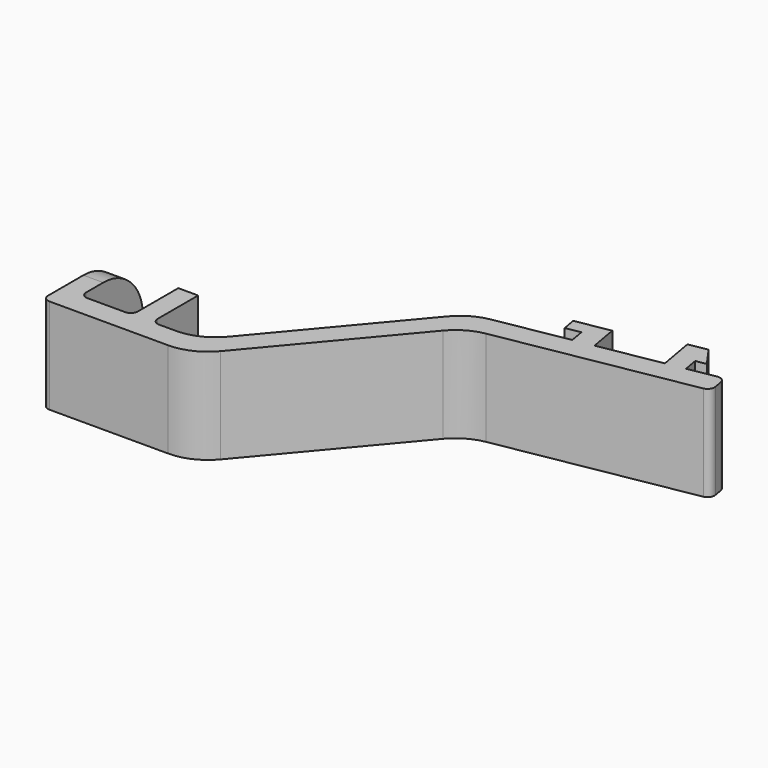
from build123d import *

# Parameters (mm, degrees)
F0_W        = 2
F0_H        = 7.85
F0_H_2      = 5.8
F1_DEPTH    = 9.6
F2_T1_DEPTH = 14.5
F3_R        = 0.7
F4_R        = 5


# Not quite as in the source:
# - a fillet or chamfer that OpenCascade refuses, or shapes differently, is made with other operations: its cross-section is extruded or revolved along the edge and cut away or added


with BuildPart() as f1:
    # F0 (on Top) → F1 (new body)
    with BuildSketch(Plane.XY):
        Polygon((-15, 0), (0, 0), (14.1413274131, 16.8529777486), (35.8070979794, 20.6732376573), (35.4077071707, 22.9382954892), (31.9608800352, 22.3305268674), (30.0897453045, 22.0005953298), (23.8854564605, 20.9066118105), (21.9158409545, 20.5593154552), (12.9175229748, 18.9726692144), (-1.0725076138, 2.3), (-5.8, 2.3), (-7.8, 2.3), (-13, 2.3), (-15, 2.3), align=None)
        with Locations((-14, 6.225)):
            Rectangle(F0_W, F0_H)
        with Locations((-6.8, 5.2)):
            Rectangle(F0_W, F0_H_2)
        Polygon((30.0897453045, 22.0005953298), (31.9608800352, 22.3305268674), (31.7004077687, 23.8077384969), (31.3183817778, 25.9743155535), (29.4472470471, 25.644384016), align=None)
        Polygon((31.3183817778, 25.9743155535), (31.7004077687, 23.8077384969), (32.7229194348, 23.9880348917), align=None)
        Polygon((21.9158409545, 20.5593154552), (23.8854564605, 20.9066118105), (23.3818767453, 23.7625542943), (21.4122612392, 23.4152579389), (21.655368688, 22.0365270847), align=None)
        Polygon((20.1781570585, 21.7760548182), (21.655368688, 22.0365270847), (21.4122612392, 23.4152579389), (19.9350496097, 23.1547856724), align=None)
    extrude(amount=F1_DEPTH)

    # F2: fillet of radius 5 on 2 edges, made by hand

    # F2_s2 → F2_t1 (cut)
    with BuildSketch(Plane.YZ.offset(-27.5)):
        with BuildLine():
            ThreePointArc((10.15, 4.6), (8.6855339059, 8.1355339059), (5.15, 9.6))
            Line((5.15, 9.6), (10.15, 9.6))
            Line((10.15, 9.6), (10.15, 4.6))
        make_face()
        with BuildLine():
            ThreePointArc((10.15, 5), (8.6855339059, 1.4644660941), (5.15, 0))
            Line((5.15, 0), (10.15, 0))
            Line((10.15, 0), (10.15, 5))
        make_face()
    extrude(amount=F2_T1_DEPTH, mode=Mode.SUBTRACT)

    # F3
    f3_edges = [f1.edges().sort_by_distance(p)[0] for p in [
        (-13, 2.3, 4.8),
        (-7.8, 2.3, 4.8),
        (-5.8, 2.3, 4.8),
        (-15, 0, 4.8),
        (35.407707, 22.938295, 4.8),
        (35.807098, 20.673238, 4.8),
    ]]
    fillet(f3_edges, radius=F3_R)

    # F4
    f4_edges = [f1.edges().sort_by_distance(p)[0] for p in [
        (0, 0, 4.8),
        (12.917523, 18.972669, 4.8),
        (14.141327, 16.852978, 4.8),
        (-1.072508, 2.3, 4.8),
    ]]
    fillet(f4_edges, radius=F4_R)


solid = f1.part
